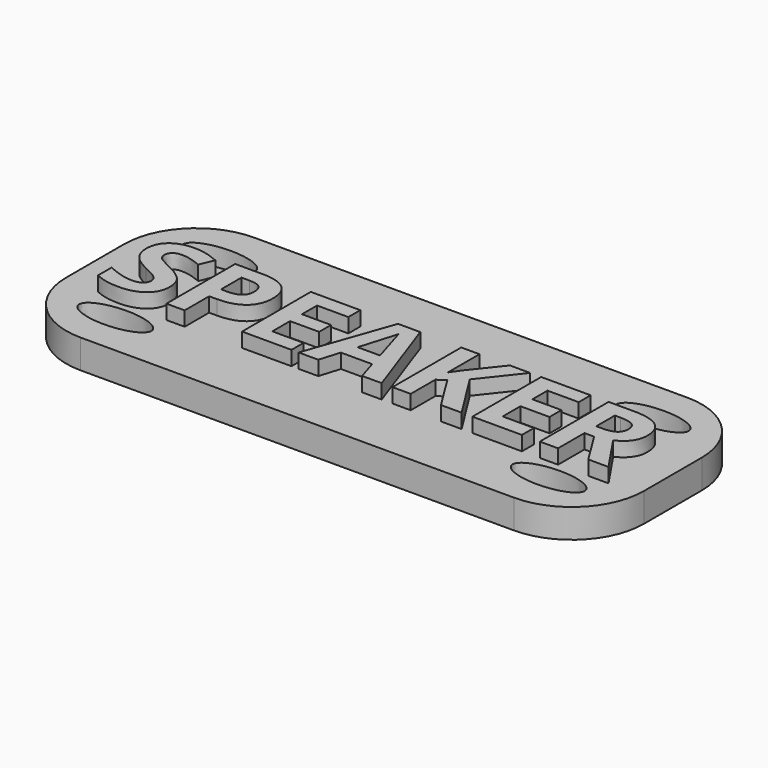
from build123d import *

# Parameters (mm, degrees)
F0_W         = 40
F0_H         = 15
F1_DEPTH     = 2
F2_TEXT_SIZE = 8.3333333333
F3_DEPTH     = 1
F4_R         = 5


# Not quite as in the source:
# - Text() gives the source's letters only with a copy of the font that has no kerning and outlines rounded to 1/6400 em; it was checked with that copy


with BuildPart() as f1:
    # F0 (on Top) → F1 (new body)
    with BuildSketch(Plane.XY):
        Rectangle(F0_W, F0_H)
        with BuildLine():
            add(Edge.make_bspline(
                [(-12.5, -4.5), (-12.5, -2.7679491924), (-16.25, -3.6339745962), (-20, -4.5), (-16.25, -5.3660254038), (-12.5, -6.2320508076), (-12.5, -4.5)],
                knots=[0, 0, 0, 2.0943951024, 2.0943951024, 4.1887902048, 4.1887902048, 6.2831853072, 6.2831853072, 6.2831853072], degree=2, weights=[1, 0.5, 1, 0.5, 1, 0.5, 1]))
        make_face(mode=Mode.SUBTRACT)
        with BuildLine():
            add(Edge.make_bspline(
                [(17.5, -4.5), (17.5, -2.7679491924), (13.75, -3.6339745962), (10, -4.5), (13.75, -5.3660254038), (17.5, -6.2320508076), (17.5, -4.5)],
                knots=[0, 0, 0, 2.0943951024, 2.0943951024, 4.1887902048, 4.1887902048, 6.2831853072, 6.2831853072, 6.2831853072], degree=2, weights=[1, 0.5, 1, 0.5, 1, 0.5, 1]))
        make_face(mode=Mode.SUBTRACT)
        with BuildLine():
            add(Edge.make_bspline(
                [(-12.5, 4.5), (-12.5, 6.2320508076), (-16.25, 5.3660254038), (-20, 4.5), (-16.25, 3.6339745962), (-12.5, 2.7679491924), (-12.5, 4.5)],
                knots=[0, 0, 0, 2.0943951024, 2.0943951024, 4.1887902048, 4.1887902048, 6.2831853072, 6.2831853072, 6.2831853072], degree=2, weights=[1, 0.5, 1, 0.5, 1, 0.5, 1]))
        make_face(mode=Mode.SUBTRACT)
        with BuildLine():
            add(Edge.make_bspline(
                [(17.5, 4.5), (17.5, 6.2320508076), (13.75, 5.3660254038), (10, 4.5), (13.75, 3.6339745962), (17.5, 2.7679491924), (17.5, 4.5)],
                knots=[0, 0, 0, 2.0943951024, 2.0943951024, 4.1887902048, 4.1887902048, 6.2831853072, 6.2831853072, 6.2831853072], degree=2, weights=[1, 0.5, 1, 0.5, 1, 0.5, 1]))
        make_face(mode=Mode.SUBTRACT)
    extrude(amount=F1_DEPTH)

    # F4
    f4_edges = [f1.edges().sort_by_distance(p)[0] for p in [
        (-20, -7.5, 1),
        (20, -7.5, 1),
        (20, 7.5, 1),
        (-20, 7.5, 1),
    ]]
    fillet(f4_edges, radius=F4_R)


with BuildPart() as f3:
    # F2 (on face) → F3 (new body)
    with BuildSketch(Plane.XY.offset(2)):
        with Locations((-18, -3)):
            Text('SPEAKER', F2_TEXT_SIZE, font='Open Sans', font_style=FontStyle.BOLD, text_align=(TextAlign.LEFT, TextAlign.BOTTOM))
    extrude(amount=F3_DEPTH)


solid = Compound([f1.part, f3.part])
